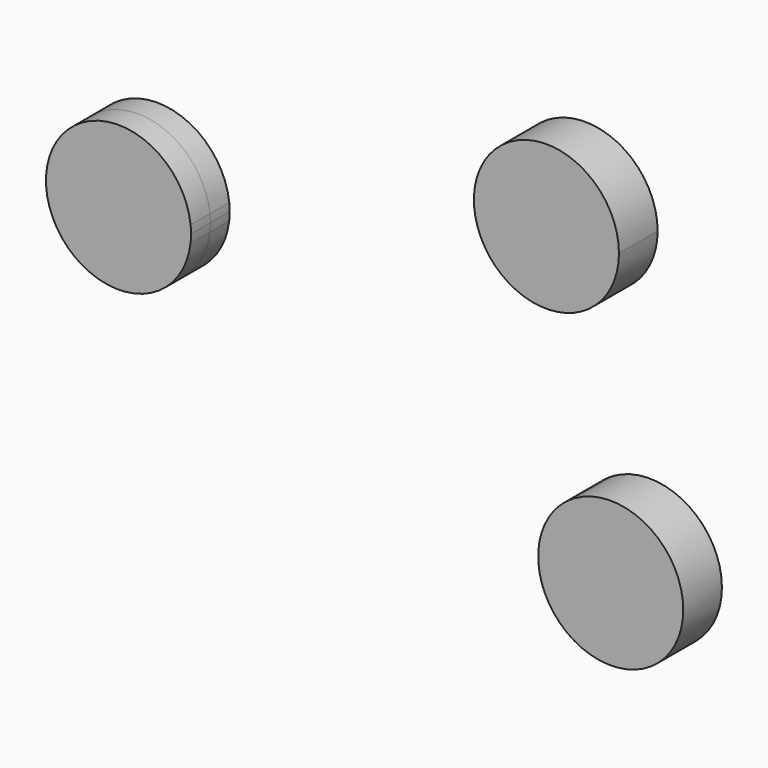
from build123d import *

# Parameters (mm, degrees)
F1_DEPTH = 6.35


with BuildPart() as f1:
    # F0 (on Front) → F1 (new body, symmetric)
    with BuildSketch(Plane.XZ):
        with BuildLine():
            ThreePointArc((40.2143343991, 36.3867283732), (54.7004476894, 41.3489042357), (60.8545334518, 55.3702414036))
            ThreePointArc((60.8545334518, 55.3702414036), (37.5758870258, 73.9449836469), (24.6318510997, 47.1239403641))
            ThreePointArc((24.6318510997, 47.1239403641), (33.2856450146, 51.1066225147), (41.8045334518, 55.3702414036))
            ThreePointArc((41.8045334518, 55.3702414036), (40.5700567026, 45.915290365), (40.2143343991, 36.3867283732))
        make_face()
        with BuildLine():
            ThreePointArc((41.8045334518, 55.3702414036), (33.2856450146, 51.1066225147), (24.6318510997, 47.1239403641))
            ThreePointArc((24.6318510997, 47.1239403641), (30.9955853075, 39.683650314), (40.2143343991, 36.3867283732))
            ThreePointArc((40.2143343991, 36.3867283732), (40.5700567026, 45.915290365), (41.8045334518, 55.3702414036))
        make_face()
    extrude(amount=F1_DEPTH, both=True)


with BuildPart() as f1b:
    # F0 (on Front) → F1, piece 2 (new body, symmetric)
    with BuildSketch(Plane.XZ):
        with BuildLine():
            ThreePointArc((77.7424552917, -21.5943939984), (68.2835676975, -5.1349571058), (49.3001389851, -5.0207132245))
            ThreePointArc((49.3001389851, -5.0207132245), (53.6126959673, -13.5249406592), (58.6924552917, -21.5943939984))
            ThreePointArc((58.6924552917, -21.5943939984), (50.6802033726, -16.4409990163), (42.4917762362, -11.572393293))
            ThreePointArc((42.4917762362, -11.572393293), (53.482869704, -39.918223238), (77.7424552917, -21.5943939984))
        make_face()
        with BuildLine():
            ThreePointArc((58.6924552917, -21.5943939984), (53.6126959673, -13.5249406592), (49.3001389851, -5.0207132245))
            ThreePointArc((49.3001389851, -5.0207132245), (45.4833114575, -7.8677403943), (42.4917762362, -11.572393293))
            ThreePointArc((42.4917762362, -11.572393293), (50.6802033726, -16.4409990163), (58.6924552917, -21.5943939984))
        make_face()
    extrude(amount=F1_DEPTH, both=True)


with BuildPart() as f1c:
    # F0 (on Front) → F1, piece 3 (new body, symmetric)
    with BuildSketch(Plane.XZ):
        with BuildLine():
            ThreePointArc((-70.5970600247, 23.2555009425), (-61.1115636291, 24.1359919206), (-51.6599442528, 25.3262849104))
            ThreePointArc((-51.6599442528, 25.3262849104), (-89.6470028775, 23.3021625557), (-51.670315931, 21.0919718782))
            ThreePointArc((-51.670315931, 21.0919718782), (-61.1146718047, 22.3400915799), (-70.5970600247, 23.2555009425))
        make_face()
        with BuildLine():
            ThreePointArc((-51.5470600247, 23.2555009425), (-51.5753020164, 24.292430194), (-51.6599442528, 25.3262849104))
            ThreePointArc((-51.6599442528, 25.3262849104), (-61.1115636291, 24.1359919206), (-70.5970600247, 23.2555009425))
            ThreePointArc((-70.5970600247, 23.2555009425), (-61.1146718047, 22.3400915799), (-51.670315931, 21.0919718782))
            ThreePointArc((-51.670315931, 21.0919718782), (-51.577898963, 22.1719823651), (-51.5470600247, 23.2555009425))
        make_face()
    extrude(amount=F1_DEPTH, both=True)


solid = Compound([f1.part, f1b.part, f1c.part])
